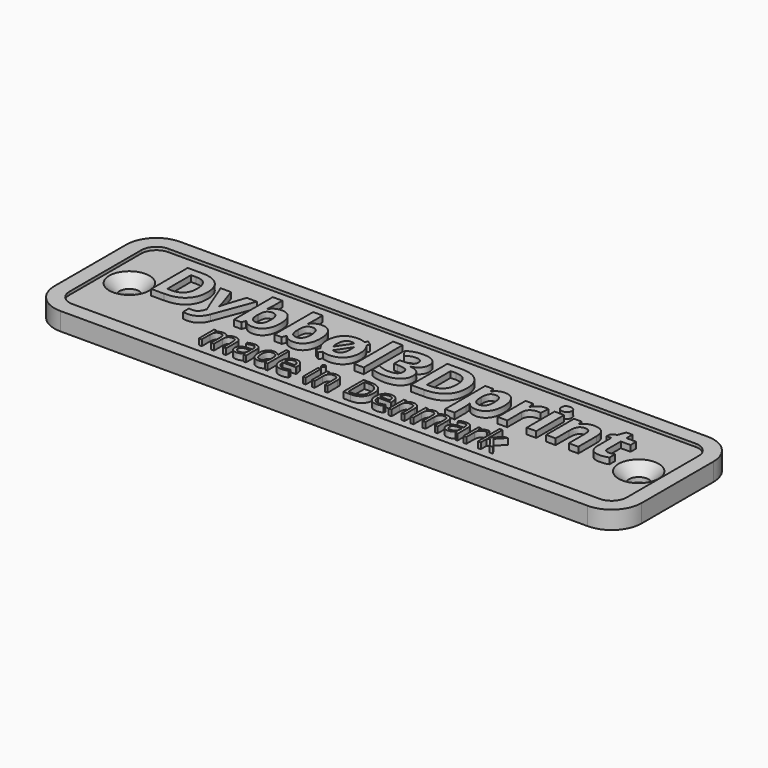
from build123d import *

# Parameters (mm, degrees)
F0_W           = 98
F0_H           = 25
F1_DEPTH       = 3
F2_R           = 5
F3_T           = -2.5
F5_D           = 3.3
F5_CSINK_D     = 6.72
F5_CSINK_ANGLE = 90
F6_TEXT_SIZE   = 10.6466473298
F6_TEXT_SIZE_2 = 5.9353785659
F7_DEPTH       = 1


# Not quite as in the source:
# - Text() gives the source's letters only with a copy of the font that has no kerning and outlines rounded to 1/6400 em; it was checked with that copy


with BuildPart() as f1:
    # F0 (on Top) → F1 (new body)
    with BuildSketch(Plane.XY):
        Rectangle(F0_W, F0_H)
    extrude(amount=F1_DEPTH)

    # F2
    f2_edges = [f1.edges().sort_by_distance(p)[0] for p in [
        (-49, -12.5, 1.5),
        (49, -12.5, 1.5),
        (49, 12.5, 1.5),
        (-49, 12.5, 1.5),
    ]]
    fillet(f2_edges, radius=F2_R)

    # F3
    f3_openings = [f1.faces().sort_by_distance(p)[0] for p in [
        (0, 0, 3),
    ]]
    offset(amount=F3_T, openings=f3_openings)

    # F5 (through all)
    with Locations(Plane.XY.offset(2.5)):
        with Locations((-42.5, 0), (42.5, 0)):
            CounterSinkHole(F5_D / 2, F5_CSINK_D / 2, counter_sink_angle=F5_CSINK_ANGLE)

    # F6 (on face) → F7 (join)
    with BuildSketch(Plane.XY.offset(2.5)):
        with Locations((-39, -1)):
            Text('Dybbøl3Dprint', F6_TEXT_SIZE, font='Open Sans', font_style=FontStyle.BOLD, text_align=(TextAlign.LEFT, TextAlign.BOTTOM))
        with Locations((-25, -8)):
            Text('made in Denmark', F6_TEXT_SIZE_2, font='Open Sans', text_align=(TextAlign.LEFT, TextAlign.BOTTOM))
    extrude(amount=F7_DEPTH)


solid = f1.part
